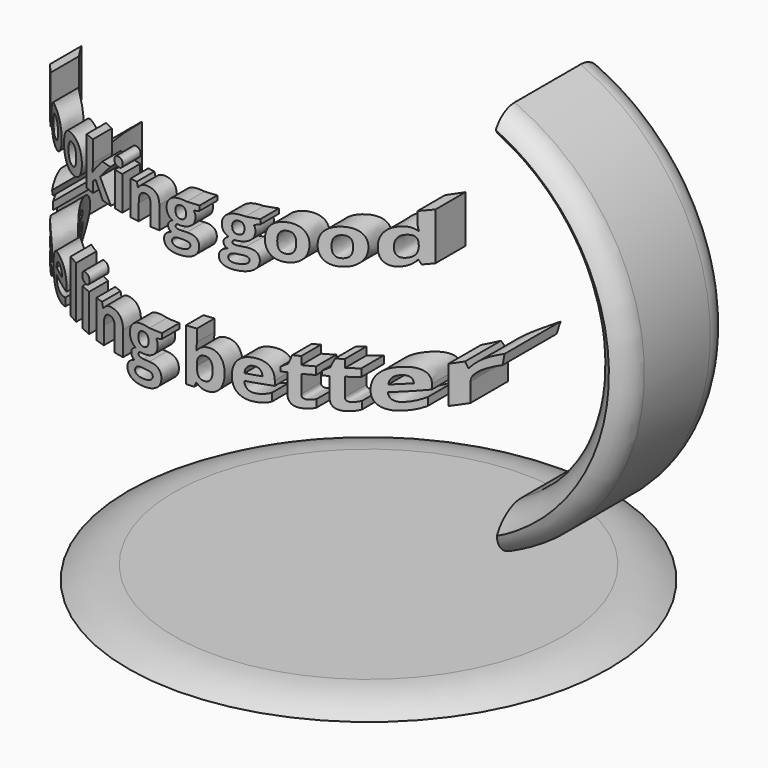
from build123d import *

# Parameters (mm, degrees)
F2_TEXT_SIZE   = 11.5252927774
F2_TEXT_SIZE_2 = 12.6229340418
F3_DEPTH       = 50.8
F6_R           = 41.91
F7_DEPTH       = 94.234
F8_R           = 44.45
F9_DEPTH       = 2.54
F12_DEPTH      = 25.4
F13_T2_ANGLE   = 168.1481252187
F13_T4_ANGLE   = 170.5408343302
F13_T6_ANGLE   = 170.5408343302
F13_T8_ANGLE   = 168.1481252187


# Not quite as in the source:
# - a fillet or chamfer that OpenCascade refuses, or shapes differently, is made with other operations: its cross-section is extruded or revolved along the edge and cut away or added
# - the program builds the solid bodies; features that only make, move or delete a surface that nothing else refers to are left out
# - Text() gives the source's letters only with a copy of the font that has no kerning and outlines rounded to 1/6400 em; it was checked with that copy


with BuildPart() as f3:
    # F2 (on Front) → F3 (new body)
    with BuildSketch(Plane.XZ):
        with Locations((-37.1097549796, 74.9071240425)):
            Text('looking good', F2_TEXT_SIZE, font='Open Sans', font_style=FontStyle.BOLD, text_align=(TextAlign.LEFT, TextAlign.BOTTOM))
        with Locations((-44.2570941523, 51.4437220991)):
            Text('feeling better', F2_TEXT_SIZE_2, font='Open Sans', font_style=FontStyle.BOLD, text_align=(TextAlign.LEFT, TextAlign.BOTTOM))
    extrude(amount=F3_DEPTH)

    # F4 (on Front) → F5 (revolve, cut)
    with BuildSketch(Plane.XZ):
        Polygon((-38.3904092014, -1.5), (-45.95, -1.5), (-45.95, 122.5), (-31.4287729561, 122.5), (-26.6426503658, 157.7727645636), (-57.9700022936, 166.4748042822), (-95.3887924552, 121.6592863202), (-111.9226738811, 52.4780452251), (-93.213275075, -4.0852311067), (-66.6720494628, -30.1913637668), (-33.6042828858, -30.1913637668), align=None)
    revolve(axis=Axis((0, 0, 93.8373953104), (0, 0, 1)), mode=Mode.SUBTRACT)

    # F6 (on Top) → F7 (cut)
    with BuildSketch(Plane.XY):
        Circle(F6_R)
    extrude(amount=F7_DEPTH, mode=Mode.SUBTRACT)


with BuildPart() as f9:
    # F8 (on Top) → F9 (new body)
    with BuildSketch(Plane.XY):
        Circle(F8_R)
    extrude(amount=F9_DEPTH)

    # F10: fillet of radius 15.3302561211 on 1 edges, made by hand

    # F10_s1 → F10_t2 (revolve, cut)
    with BuildSketch(Plane.XZ):
        with BuildLine():
            ThreePointArc((44.45, 0), (40.4110207699, 1.8912740262), (35.9986036009, 2.54))
            Line((35.9986036009, 2.54), (44.45, 2.54))
            Line((44.45, 2.54), (44.45, 0))
        make_face()
    revolve(axis=Axis((0, 0, 2.54), (0, 0, 1)), mode=Mode.SUBTRACT)


with BuildPart() as f12:
    # F11 (on Front) → F12 (new body)
    with BuildSketch(Plane.XZ):
        with BuildLine():
            ThreePointArc((43.269213289, 94.5153683424), (61.4578747609, 65.6307415284), (44.4546714425, 36.0327661037))
            Line((44.4546714425, 36.0327661037), (43.269213289, 27.3521318935))
            ThreePointArc((43.269213289, 27.3521318935), (67.2520634628, 63.6934535578), (43.269213289, 100.0347752221))
            Line((43.269213289, 100.0347752221), (43.269213289, 94.5153683424))
        make_face()
    extrude(amount=F12_DEPTH)

    # F13: fillet of radius 5.08 on 4 edges, made by hand

    # F13_s1 → F13_t2 (revolve, cut)
    with BuildSketch(Plane(origin=(22.7901320082, 0, -1.899599738), x_dir=(0, 1, 0), z_dir=(-0.9965442307, 0, 0.0830638084))):
        with BuildLine():
            ThreePointArc((-20.32, -100.1930293191), (-23.9121024484, -101.6809268707), (-25.4, -105.2730293191))
            Line((-25.4, -105.2730293191), (-25.4, -100.1930293191))
            Line((-25.4, -100.1930293191), (-20.32, -100.1930293191))
        make_face()
    revolve(axis=Axis((28.3629951645, -25.4, 64.9598993744), (0, 1, 0)), revolution_arc=F13_T2_ANGLE, mode=Mode.SUBTRACT)

    # F13_s3 → F13_t4 (revolve, cut)
    with BuildSketch(Plane(origin=(32.7718933233, 0, 2.7113758984), x_dir=(0, 1, 0), z_dir=(-0.9965949477, 0, -0.0824530794))):
        with BuildLine():
            ThreePointArc((-20.32, -21.6649244155), (-23.9121024484, -23.152821967), (-25.4, -26.7449244155))
            Line((-25.4, -26.7449244155), (-25.4, -21.6649244155))
            Line((-25.4, -21.6649244155), (-20.32, -21.6649244155))
        make_face()
    revolve(axis=Axis((27.7265535874, -25.4, 63.6934535578), (0, -1, 0)), revolution_arc=F13_T4_ANGLE, mode=Mode.SUBTRACT)

    # F13_s5 → F13_t6 (revolve, cut)
    with BuildSketch(Plane(origin=(32.7718933233, 0, 2.7113758984), x_dir=(0, 1, 0), z_dir=(-0.9965949477, 0, -0.0824530794))):
        with BuildLine():
            ThreePointArc((-5.08, -21.6649244155), (-1.4878975516, -23.152821967), (0, -26.7449244155))
            Line((0, -26.7449244155), (0, -21.6649244155))
            Line((0, -21.6649244155), (-5.08, -21.6649244155))
        make_face()
    revolve(axis=Axis((27.7265535874, 0, 63.6934535578), (0, -1, 0)), revolution_arc=F13_T6_ANGLE, mode=Mode.SUBTRACT)

    # F13_s7 → F13_t8 (revolve, cut)
    with BuildSketch(Plane(origin=(22.7901320082, 0, -1.899599738), x_dir=(0, 1, 0), z_dir=(-0.9965442307, 0, 0.0830638084))):
        with BuildLine():
            ThreePointArc((-5.08, -100.1930293191), (-1.4878975516, -101.6809268707), (0, -105.2730293191))
            Line((0, -105.2730293191), (0, -100.1930293191))
            Line((0, -100.1930293191), (-5.08, -100.1930293191))
        make_face()
    revolve(axis=Axis((28.3629951645, 0, 64.9598993744), (0, 1, 0)), revolution_arc=F13_T8_ANGLE, mode=Mode.SUBTRACT)


solid = Compound([f3.part, f9.part, f12.part])
